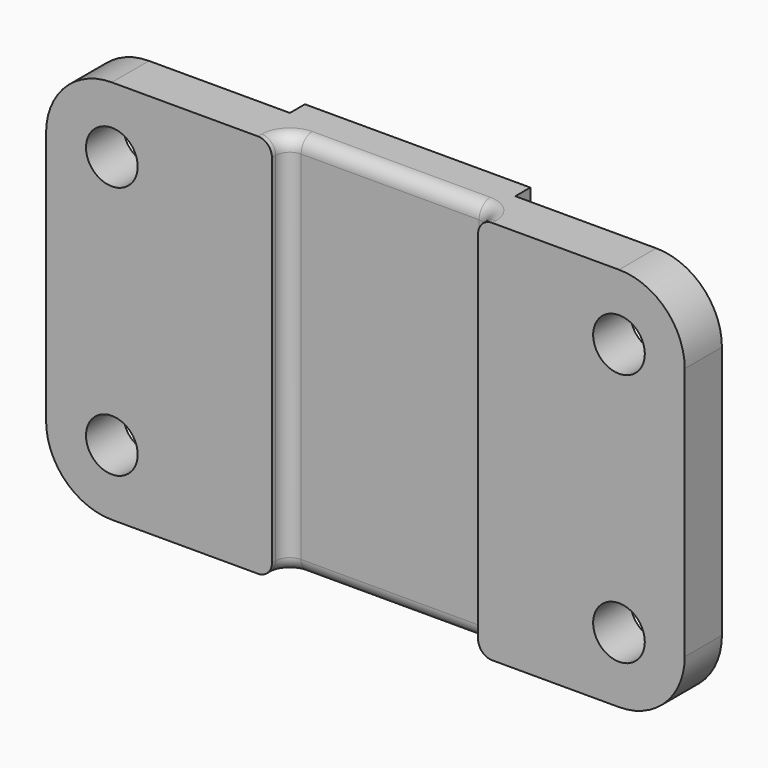
from build123d import *

# Parameters (mm, degrees)
F0_W     = 48
F0_H     = 82
F1_DEPTH = 4
F0_R     = 5.5
F2_DEPTH = 9.9
F3_W     = 43.8994949366
F3_H     = 82
F4_DEPTH = 4
F5_F1_R  = 3
F5_F2_R  = 3


with BuildPart() as f1:
    # F0 (on Front) → F1 (new body)
    with BuildSketch(Plane.XZ):
        with Locations((68, 41)):
            Rectangle(F0_W, F0_H)
    extrude(amount=-F1_DEPTH)

    # F0 (on Front) → F2 (join)
    with BuildSketch(Plane.XZ):
        with BuildLine():
            ThreePointArc((0, 14), (4.1005050634, 4.1005050634), (14, 0))
            Line((14, 0), (44, 0))
            Line((44, 0), (44, 82))
            Line((44, 82), (14, 82))
            ThreePointArc((14, 82), (4.1005050634, 77.8994949366), (0, 68))
            Line((0, 68), (0, 14))
        make_face()
        with Locations((14, 14)):
            Circle(F0_R, mode=Mode.SUBTRACT)
        with Locations((14, 68)):
            Circle(F0_R, mode=Mode.SUBTRACT)
        with Locations((68, 41)):
            Rectangle(F0_W, F0_H)
        with BuildLine():
            Line((92, 82), (92, 0))
            Line((92, 0), (122, 0))
            ThreePointArc((122, 0), (131.8994949366, 4.1005050634), (136, 14))
            Line((136, 14), (136, 68))
            ThreePointArc((136, 68), (131.8994949366, 77.8994949366), (122, 82))
            Line((122, 82), (92, 82))
        make_face()
        with Locations((122, 14)):
            Circle(F0_R, mode=Mode.SUBTRACT)
        with Locations((122, 68)):
            Circle(F0_R, mode=Mode.SUBTRACT)
    extrude(amount=F2_DEPTH)

    # F3 (on face) → F4 (cut)
    with BuildSketch(Plane.XZ.offset(9.9)):
        with Locations((70.0502525317, 41)):
            Rectangle(F3_W, F3_H)
    extrude(amount=-F4_DEPTH, mode=Mode.SUBTRACT)

    # F5: fillet of radius 3 on 4 edges, made by hand

    # F5_f1
    f5_f1_edges = [f1.edges().sort_by_distance(p)[0] for p in [
        (48.1005050634, -5.9, 41),
        (92, -5.9, 41),
    ]]
    fillet(f5_f1_edges, radius=F5_F1_R)

    # F5_f2
    f5_f2_edges = [f1.edges().sort_by_distance(p)[0] for p in [
        (70.0502525317, -5.9, 0),
        (70.0502525317, -5.9, 82),
        (91.1213203436, -6.7786796564, 82),
        (48.9791847198, -6.7786796564, 82),
        (48.9791847198, -6.7786796564, 0),
        (91.1213203436, -6.7786796564, 0),
    ]]
    fillet(f5_f2_edges, radius=F5_F2_R)


solid = f1.part
